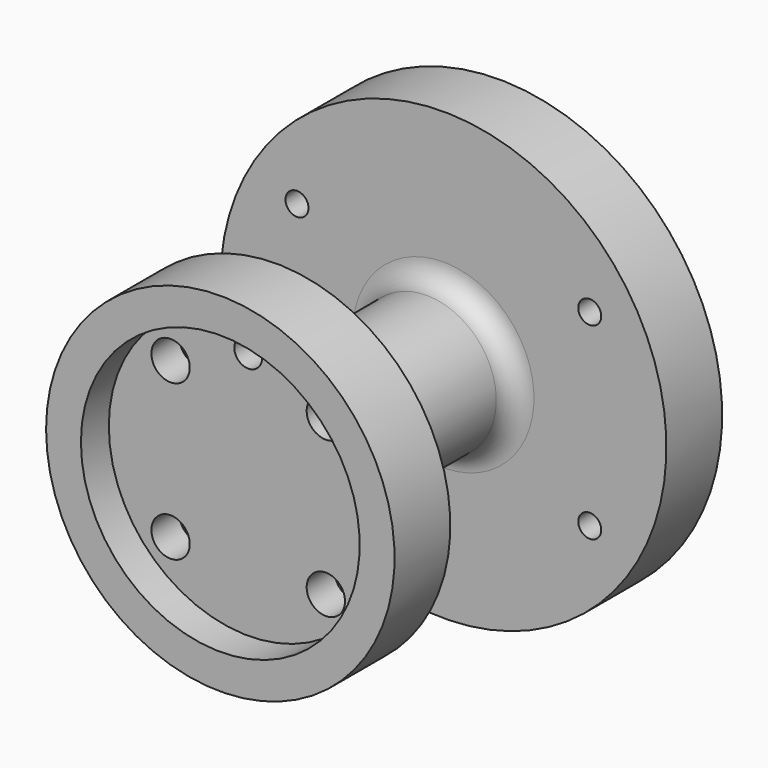
from build123d import *

# Parameters (mm, degrees)
F3_D            = 3.3
F3_DEPTH        = 14.1
F3_TIP          = 0.9914200214
F2_R            = 4
F4_DEPTH        = 3
F5_R            = 2.75
F6_DEPTH        = 25
F6_COPIES_COUNT = 4
F8_R            = 2
F9_DEPTH        = 25


# Not quite as in the source:
# - a pattern or mirror of a feature is missing from the dataset's text; its kind, count and spacing are read off the source's solid


with BuildPart() as f1:
    # F0 (on Top) → F1 (revolve)
    with BuildSketch(Plane.XY):
        with BuildLine():
            Line((-25, 0), (-20, 0))
            Line((-20, 0), (-20, 5))
            Line((-20, 5), (0, 5))
            Line((0, 5), (0, 50))
            Line((0, 50), (-32, 50))
            Line((-32, 50), (-32, 40))
            Line((-32, 40), (-13, 40))
            ThreePointArc((-13, 40), (-10.8786796564, 39.1213203436), (-10, 37))
            Line((-10, 37), (-10, 13))
            ThreePointArc((-10, 13), (-10.8786796564, 10.8786796564), (-13, 10))
            Line((-13, 10), (-25, 10))
            Line((-25, 10), (-25, 0))
        make_face()
    revolve(axis=Axis((0, 27.5, 0), (0, -1, 0)))

    # F3
    with Locations(Plane(origin=(0, 50, 0), x_dir=(-1, 0, 0), z_dir=(0, 1, 0))):
        with Locations((21, -13.5), (21, 13.5), (-21, 13.5), (-21, -13.5)):
            Hole(F3_D / 2, depth=F3_DEPTH)
            with Locations((0, 0, -(F3_DEPTH + F3_TIP / 2))):  # 118° drill point
                Cone(0, F3_D / 2, F3_TIP, mode=Mode.SUBTRACT)

    # F2 (on face) → F4 (cut)
    with BuildSketch(Plane(origin=(0, 50, 0), x_dir=(-1, 0, 0), z_dir=(0, 1, 0))):
        with Locations((21, -13.5)):
            Circle(F2_R)
        with Locations((-21, 13.5)):
            Circle(F2_R)
    extrude(amount=-F4_DEPTH, mode=Mode.SUBTRACT)

    # F5 (on face) → F6 (cut)
    with BuildSketch(Plane.XZ.offset(-5)):
        with Locations((11.1369318037, -11.1369318037)):
            Circle(F5_R)
    f6 = extrude(amount=-F6_DEPTH, mode=Mode.SUBTRACT)

    # F6_copies: F6 ×4 about axis
    f6_copies_axis = Axis((0, 0, 0), (0, 1, 0))
    for i in range(1, F6_COPIES_COUNT):
        add(f6.rotate(f6_copies_axis, i * 360 / F6_COPIES_COUNT), mode=Mode.SUBTRACT)

    # F8 (on face) → F9 (cut)
    with BuildSketch(Plane.XZ.offset(-5)):
        with Locations((0, 15.75)):
            Circle(F8_R)
    extrude(amount=-F9_DEPTH, mode=Mode.SUBTRACT)


solid = f1.part
